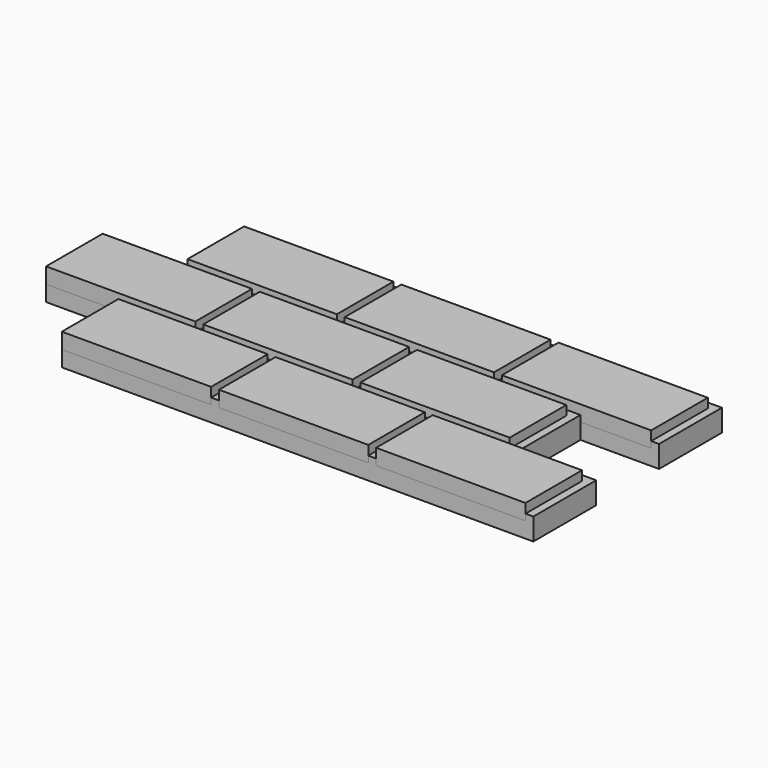
from build123d import *

# Parameters (mm, degrees)
F1_DEPTH = 20
F2_W     = 190
F2_H     = 90
F3_DEPTH = 20
F4_W     = 190
F4_H     = 90
F5_DEPTH = 8


with BuildPart() as f1:
    # F0 (on Top) → F1 (new body)
    with BuildSketch(Plane.XY):
        Polygon((-250, -150), (350, -150), (350, -50), (250, -50), (250, 50), (350, 50), (350, 150), (-250, 150), (-250, 50), (-350, 50), (-350, -50), (-250, -50), align=None)
    extrude(amount=F1_DEPTH)

    # F4 (on face) → F5 (join)
    with BuildSketch(Plane.XY.offset(20)):
        Polygon((350, 50), (350, 150), (-250, 150), (-250, 140), (-60, 140), (-60, 50), (-250, 50), (-350, 50), (-350, 40), (-160, 40), (-160, -50), (-250, -50), (-250, -60), (-60, -60), (-60, -150), (-50, -150), (-50, -60), (140, -60), (140, -150), (150, -150), (150, -60), (340, -60), (340, -150), (350, -150), (350, -50), (250, -50), (250, 50), (150, 50), (150, 140), (340, 140), (340, 50), align=None)
        with Locations((-55, -5)):
            Rectangle(F4_W, F4_H, mode=Mode.SUBTRACT)
        with Locations((145, -5)):
            Rectangle(F4_W, F4_H, mode=Mode.SUBTRACT)
        with Locations((45, 95)):
            Rectangle(F4_W, F4_H, mode=Mode.SUBTRACT)
    extrude(amount=F5_DEPTH)


with BuildPart() as f3:
    # F2 (on face) → F3 (new body)
    with BuildSketch(Plane.XY.offset(20)):
        with Locations((-255, -5)):
            Rectangle(F2_W, F2_H)
    extrude(amount=F3_DEPTH)


with BuildPart() as f3b:
    # F2 (on face) → F3, piece 2 (new body)
    with BuildSketch(Plane.XY.offset(20)):
        with Locations((-55, -5)):
            Rectangle(F2_W, F2_H)
    extrude(amount=F3_DEPTH)


with BuildPart() as f3c:
    # F2 (on face) → F3, piece 3 (new body)
    with BuildSketch(Plane.XY.offset(20)):
        with Locations((145, -5)):
            Rectangle(F2_W, F2_H)
    extrude(amount=F3_DEPTH)


with BuildPart() as f3d:
    # F2 (on face) → F3, piece 4 (new body)
    with BuildSketch(Plane.XY.offset(20)):
        with Locations((-155, 95)):
            Rectangle(F2_W, F2_H)
    extrude(amount=F3_DEPTH)


with BuildPart() as f3e:
    # F2 (on face) → F3, piece 5 (new body)
    with BuildSketch(Plane.XY.offset(20)):
        with Locations((45, 95)):
            Rectangle(F2_W, F2_H)
    extrude(amount=F3_DEPTH)


with BuildPart() as f3f:
    # F2 (on face) → F3, piece 6 (new body)
    with BuildSketch(Plane.XY.offset(20)):
        with Locations((245, 95)):
            Rectangle(F2_W, F2_H)
    extrude(amount=F3_DEPTH)


with BuildPart() as f3g:
    # F2 (on face) → F3, piece 7 (new body)
    with BuildSketch(Plane.XY.offset(20)):
        with Locations((-155, -105)):
            Rectangle(F2_W, F2_H)
    extrude(amount=F3_DEPTH)


with BuildPart() as f3h:
    # F2 (on face) → F3, piece 8 (new body)
    with BuildSketch(Plane.XY.offset(20)):
        with Locations((45, -105)):
            Rectangle(F2_W, F2_H)
    extrude(amount=F3_DEPTH)


with BuildPart() as f3i:
    # F2 (on face) → F3, piece 9 (new body)
    with BuildSketch(Plane.XY.offset(20)):
        with Locations((245, -105)):
            Rectangle(F2_W, F2_H)
    extrude(amount=F3_DEPTH)


solid = Compound([f1.part, f3.part, f3b.part, f3c.part, f3d.part, f3e.part, f3f.part, f3g.part, f3h.part, f3i.part])
